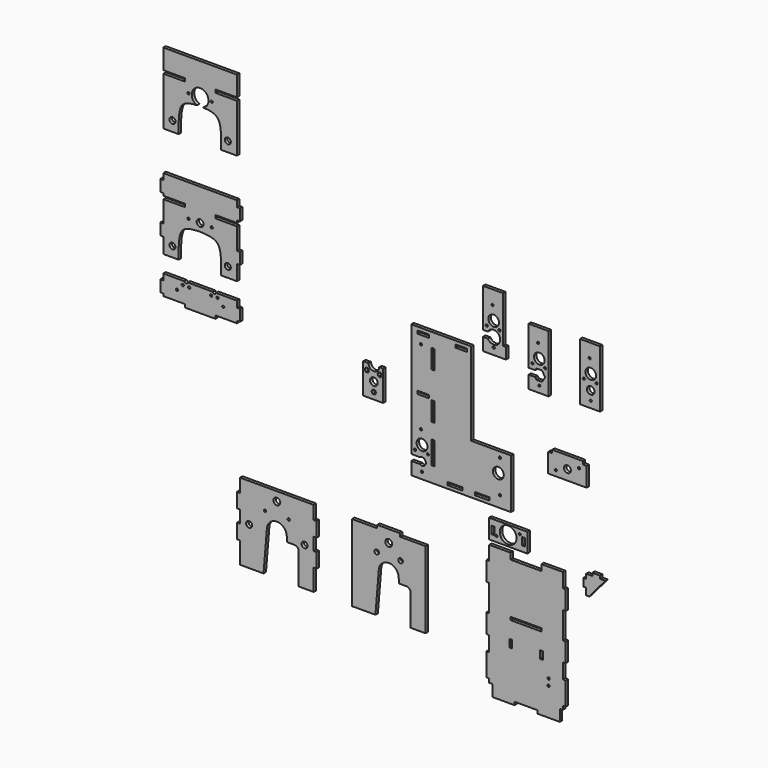
from build123d import *

# Parameters (mm, degrees)
F0_R      = 1.4
F0_R_2    = 7.1
F0_W      = 3.9
F0_H      = 30
F0_W_2    = 19
F0_H_2    = 3.9
F0_H_3    = 25
F0_R_3    = 1.5
F0_W_3    = 15
F2_DEPTH  = 4
F1_R      = 1.4
F1_R_2    = 4.5
F3_DEPTH  = 4
F4_R      = 1.4
F4_W      = 3.9
F4_H      = 10
F4_R_2    = 10.9
F5_DEPTH  = 4
F7_DEPTH  = 4
F8_W      = 3.7
F8_H      = 10
F8_R      = 1.5
F8_W_2    = 40
F8_H_2    = 3.9
F9_DEPTH  = 4
F10_R     = 1.4
F10_R_2   = 6.95
F11_DEPTH = 4
F12_R     = 1.5
F12_R_2   = 1.4
F12_R_3   = 6.95
F13_DEPTH = 4
F14_R     = 1.4
F14_R_2   = 5
F14_R_3   = 6.95
F15_DEPTH = 4
F16_R     = 5
F17_DEPTH = 4
F18_R     = 3
F18_R_2   = 4.5
F19_DEPTH = 4
F20_R     = 3.925
F20_R_2   = 1.5
F20_R_3   = 4.5
F21_DEPTH = 4
F22_R     = 1.45
F22_R_2   = 1.5
F23_DEPTH = 4
F24_R     = 3.925
F24_R_2   = 1.4
F24_R_3   = 4.5
F25_DEPTH = 4
F26_R     = 3.925
F26_R_2   = 1.4
F27_DEPTH = 4


# Not quite as in the source:
# - ends of sketch curves that miss each other by under 0.0002 mm in the source are joined
# - the dataset's text gives a spline's control points without its knots; the knots are read off the source's solid


with BuildPart() as f2:
    # F0 (on Front) → F2 (new body)
    with BuildSketch(Plane.XZ):
        with BuildLine():
            Line((-63.4341964287, 90.4360366771), (-63.4341964287, -22.9460053229))
            Line((-63.4341964287, -22.9460053229), (-63.4341964287, -58.4452043229))
            Line((-63.4341964287, -58.4452043229), (-52.4341964287, -58.4452043229))
            ThreePointArc((-52.4341964287, -58.4452043229), (-47.1981284512, -57.9730683679), (-44.4341964287, -62.4452043229))
            ThreePointArc((-44.4341964287, -62.4452043229), (-47.1981284512, -66.9173402779), (-52.4341964287, -66.4452043229))
            Line((-52.4341964287, -66.4452043229), (-63.4341964287, -66.4452043229))
            Line((-63.4341964287, -66.4452043229), (-63.4341964287, -82.9460053229))
            Line((-63.4341964287, -82.9460053229), (66.5658035713, -82.9460053229))
            Line((66.5658035713, -82.9460053229), (66.5629615713, -50.5350533229))
            Line((66.5629615713, -50.5350533229), (66.5658035713, -17.9460053229))
            Line((66.5658035713, -17.9460053229), (29.5658035713, -17.9460053229))
            Line((29.5658035713, -17.9460053229), (19.5658035713, -17.9460053229))
            Line((19.5658035713, -17.9460053229), (14.5658035713, -17.9460053229))
            Line((14.5658035713, -17.9460053229), (14.5658035713, 90.4360366771))
            Line((14.5658035713, 90.4360366771), (-63.4341964287, 90.4360366771))
        make_face()
        with Locations((-49.4341964287, -74.3492573229)):
            Circle(F0_R, mode=Mode.SUBTRACT)
        with Locations((-58.4986314287, -51.9228453229)):
            Circle(F0_R, mode=Mode.SUBTRACT)
        with Locations((-49.4341964287, -43.4452043229)):
            Circle(F0_R_2, mode=Mode.SUBTRACT)
        with Locations((-41.8097264287, -51.9228453229)):
            Circle(F0_R, mode=Mode.SUBTRACT)
        with Locations((-35.4341964287, -47.9460053229)):
            Rectangle(F0_W, F0_H, mode=Mode.SUBTRACT)
        with Locations((-6.4341964287, -76.9460053229)):
            Rectangle(F0_W_2, F0_H_2, mode=Mode.SUBTRACT)
        with Locations((-50.9341964287, -25.9460053229)):
            Circle(F0_R, mode=Mode.SUBTRACT)
        with Locations((-35.4341964287, -0.4460053229)):
            Rectangle(F0_W, F0_H_3, mode=Mode.SUBTRACT)
        with Locations((29.0658035713, -76.9460053229)):
            Rectangle(F0_W_2, F0_H_2, mode=Mode.SUBTRACT)
        with Locations((52.2136285713, -67.9460053229)):
            Circle(F0_R_3, mode=Mode.SUBTRACT)
        with Locations((50.0757545713, -43.5444653229)):
            Circle(F0_R_2, mode=Mode.SUBTRACT)
        with Locations((52.2136285713, -24.9473123229)):
            Circle(F0_R_3, mode=Mode.SUBTRACT)
        with Locations((-47.9341964287, 14.9539946771)):
            Rectangle(F0_W_3, F0_H_2, mode=Mode.SUBTRACT)
        with Locations((-35.4341964287, 59.5539946771)):
            Rectangle(F0_W, F0_H_3, mode=Mode.SUBTRACT)
        with Locations((-50.9341964287, 71.6313536771)):
            Circle(F0_R, mode=Mode.SUBTRACT)
        with Locations((-47.9341964287, 84.2463486771)):
            Rectangle(F0_W_3, F0_H_2, mode=Mode.SUBTRACT)
        with Locations((1.9138515713, 84.2463486771)):
            Rectangle(F0_W_3, F0_H_2, mode=Mode.SUBTRACT)
    extrude(amount=F2_DEPTH)


with BuildPart() as f3:
    # F1 (on Front) → F3 (new body)
    with BuildSketch(Plane.XZ):
        Polygon((115.1583404474, -22.8264850692), (120.1583404474, -22.8264850692), (160.1583404474, -22.8264850692), (165.1583404474, -22.8264850692), (165.1583404474, 2.1735149308), (162.1583404474, 2.1735149308), (160.1583404474, 2.1735149308), (160.1583404474, 6.1735149308), (120.1583404474, 6.1735149308), (120.1583404474, 2.1735149308), (118.1583404474, 2.1735149308), (115.1583404474, 2.1735149308), (115.1583404474, -9.8264850692), align=None)
        with Locations((124.9870464474, -15.6336020692)):
            Circle(F1_R, mode=Mode.SUBTRACT)
        with Locations((140.1583404474, -9.6756990692)):
            Circle(F1_R_2, mode=Mode.SUBTRACT)
        with Locations((155.3296344474, -3.7691630692)):
            Circle(F1_R, mode=Mode.SUBTRACT)
    extrude(amount=F3_DEPTH)


with BuildPart() as f5:
    # F4 (on Front) → F5 (new body)
    with BuildSketch(Plane.XZ):
        Polygon((82.8902986646, -98.5648238522), (42.8902986646, -98.5648238522), (37.8902986646, -98.5648238522), (37.8902986646, -110.5648238522), (37.8902986646, -123.5648238522), (42.8902986646, -123.5648238522), (82.8902986646, -123.5648238522), (87.8902986646, -123.5648238522), (87.8902986646, -110.5648238522), (87.8902986646, -98.5648238522), align=None)
        with Locations((47.7190046646, -116.3719408522)):
            Circle(F4_R, mode=Mode.SUBTRACT)
        with Locations((42.9902986646, -111.5648238522)):
            Rectangle(F4_W, F4_H, mode=Mode.SUBTRACT)
        with Locations((82.7902986646, -111.5648238522)):
            Rectangle(F4_W, F4_H, mode=Mode.SUBTRACT)
        with Locations((62.8902986646, -110.4140378522)):
            Circle(F4_R_2, mode=Mode.SUBTRACT)
        with Locations((78.0615926646, -104.5075018522)):
            Circle(F4_R, mode=Mode.SUBTRACT)
    extrude(amount=F5_DEPTH)


with BuildPart() as f7:
    # F6 (on Front) → F7 (new body)
    with BuildSketch(Plane.XZ):
        Polygon((164.545552, -137.732495), (164.545552, -146.610202), (168.63066, -146.610202), (189.545552, -121.732495), (182.545552, -121.732495), (182.545552, -118.032495), (172.545552, -118.032495), (172.545552, -121.732495), (164.545552, -121.732495), (164.545552, -127.732495), (160.845552, -127.732495), (160.845552, -137.732495), align=None)
    extrude(amount=F7_DEPTH)


with BuildPart() as f9:
    # F8 (on Front) → F9 (new body)
    with BuildSketch(Plane.XZ):
        Polygon((134.185844, -129.659568), (106.185844, -129.659568), (106.185844, -137.659568), (66.185844, -137.659568), (66.185844, -129.659568), (38.185844, -129.659568), (38.185844, -148.305989), (34.485844, -148.305989), (34.485844, -173.305989), (38.185844, -173.305989), (38.185844, -208.305989), (34.485844, -208.305989), (34.485844, -233.305989), (38.185844, -233.305989), (38.185844, -253.04161), (34.485844, -253.04161), (34.485844, -283.04161), (38.185844, -283.04161), (38.185844, -288.04161), (42.185844, -288.04161), (42.185844, -303.04161), (71.185844, -303.04161), (71.185844, -299.04161), (101.185844, -299.04161), (101.185844, -303.04161), (130.185844, -303.04161), (130.185844, -288.04161), (134.185844, -288.04161), (134.185844, -283.04161), (137.885844, -283.04161), (137.885844, -253.04161), (134.185844, -253.04161), (134.185844, -233.305989), (137.885844, -233.305989), (137.885844, -208.305989), (134.185844, -208.305989), (134.185844, -173.305989), (137.885844, -173.305989), (137.885844, -148.305989), (134.185844, -148.305989), align=None)
        with Locations((66.166966, -234.041521)):
            Rectangle(F8_W, F8_H, mode=Mode.SUBTRACT)
        with Locations((115.552706, -266.295691)):
            Circle(F8_R, mode=Mode.SUBTRACT)
        Polygon((108.016966, -229.041521), (108.016966, -239.041521), (104.316966, -239.041521), (104.316966, -229.084858), (104.316966, -229.041521), align=None, mode=Mode.SUBTRACT)
        with Locations((115.552706, -257.951092)):
            Circle(F8_R, mode=Mode.SUBTRACT)
        with Locations((86.185844, -205.14161)):
            Rectangle(F8_W_2, F8_H_2, mode=Mode.SUBTRACT)
    extrude(amount=F9_DEPTH)


with BuildPart() as f11:
    # F10 (on Front) → F11 (new body)
    with BuildSketch(Plane.XZ):
        Polygon((89.4677672969, 81.3291730556), (89.4677672969, 65.8326860556), (115.5677672969, 65.8326860556), (115.5677672969, 140.8326860556), (89.4677672969, 140.8326860556), (89.4677672969, 90.3228060556), (98.2716152969, 90.3228060556), (99.7149902969, 92.8228060556), (107.2205442969, 92.8228060556), (110.9733212969, 86.3228060556), (107.2205442969, 79.8228060556), (99.7149902969, 79.8228060556), (98.2716150084, 82.322805889), (89.4677672969, 82.3228060556), align=None)
        with Locations((94.4033322969, 96.8451650556)):
            Circle(F10_R, mode=Mode.SUBTRACT)
        with Locations((103.4677672969, 74.4187530556)):
            Circle(F10_R, mode=Mode.SUBTRACT)
        with Locations((111.0922382969, 96.8451650556)):
            Circle(F10_R, mode=Mode.SUBTRACT)
        with Locations((101.9677672969, 122.8326860556)):
            Circle(F10_R, mode=Mode.SUBTRACT)
        with Locations((103.4677672969, 105.3228060556)):
            Circle(F10_R_2, mode=Mode.SUBTRACT)
    extrude(amount=F11_DEPTH)


with BuildPart() as f13:
    # F12 (on Front) → F13 (new body)
    with BuildSketch(Plane.XZ):
        with BuildLine():
            Line((30.0127932642, 106.5112202716), (30.0127932642, 90.0211002716))
            Line((30.0127932642, 90.0211002716), (60.0127932642, 90.0211002716))
            Line((60.0127932642, 90.0211002716), (60.0127932642, 104.5211002716))
            Line((60.0127932642, 104.5211002716), (56.1127932642, 104.5211002716))
            Line((56.1127932642, 104.5211002716), (56.1127932642, 165.0211002716))
            Line((56.1127932642, 165.0211002716), (30.0127932642, 165.0211002716))
            Line((30.0127932642, 165.0211002716), (30.0127932642, 114.5112202716))
            Line((30.0127932642, 114.5112202716), (36.5127932642, 114.5112202716))
            ThreePointArc((36.5127932642, 114.5112202716), (46.0743460771, 118.7574315228), (52.5127932642, 110.5112202716))
            ThreePointArc((52.5127932642, 110.5112202716), (46.0743460771, 102.2650090204), (36.5127932642, 106.5112202716))
            Line((36.5127932642, 106.5112202716), (30.0127932642, 106.5112202716))
        make_face()
        with Locations((44.0127932642, 98.6071672716)):
            Circle(F12_R, mode=Mode.SUBTRACT)
        with Locations((34.9483582642, 121.0335792716)):
            Circle(F12_R_2, mode=Mode.SUBTRACT)
        with Locations((44.0127932642, 129.5112202716)):
            Circle(F12_R_3, mode=Mode.SUBTRACT)
        with Locations((42.5127932642, 147.0211002716)):
            Circle(F12_R_2, mode=Mode.SUBTRACT)
        with Locations((51.6372632642, 121.0335792716)):
            Circle(F12_R_2, mode=Mode.SUBTRACT)
    extrude(amount=F13_DEPTH)


with BuildPart() as f15:
    # F14 (on Front) → F15 (new body)
    with BuildSketch(Plane.XZ):
        Polygon((156.5812625652, 109.6729690981), (156.5812625652, 70.1828490981), (182.6812625652, 70.1828490981), (182.6812625652, 84.6828490981), (182.6812625652, 109.6729690981), (182.6812625652, 145.1828490981), (156.5812625652, 145.1828490981), align=None)
        with Locations((161.5168275652, 101.1953280981)):
            Circle(F14_R, mode=Mode.SUBTRACT)
        with Locations((170.5812625652, 78.7689160981)):
            Circle(F14_R, mode=Mode.SUBTRACT)
        with Locations((170.5812625652, 90.6729690981)):
            Circle(F14_R_2, mode=Mode.SUBTRACT)
        with Locations((178.2057335652, 101.1953280981)):
            Circle(F14_R, mode=Mode.SUBTRACT)
        with Locations((169.0812625652, 127.1828490981)):
            Circle(F14_R, mode=Mode.SUBTRACT)
        with Locations((170.5812625652, 109.6729690981)):
            Circle(F14_R_3, mode=Mode.SUBTRACT)
    extrude(amount=F15_DEPTH)


with BuildPart() as f17:
    # F16 (on Front) → F17 (new body)
    with BuildSketch(Plane.XZ):
        with BuildLine():
            Line((-126.2313253517, 27.6353715188), (-126.2313253517, -11.8547484812))
            Line((-126.2313253517, -11.8547484812), (-100.1313253517, -11.8547484812))
            Line((-100.1313253517, -11.8547484812), (-100.1313253517, 27.6353715188))
            Line((-100.1313253517, 27.6353715188), (-105.2813253517, 27.6353715188))
            ThreePointArc((-105.2813253517, 27.6353715188), (-112.2313253517, 20.6853715188), (-119.1813253517, 27.6353715188))
            Line((-119.1813253517, 27.6353715188), (-126.2313253517, 27.6353715188))
        make_face()
        Polygon((-113.7540863517, -0.6311814812), (-110.7085633517, -0.6311814812), (-109.1858023517, -3.2686814812), (-110.7085633517, -5.9061814812), (-113.7540863517, -5.9061814812), (-115.2768473517, -3.2686814812), align=None, mode=Mode.SUBTRACT)
        Polygon((-122.8185213517, 21.7952305188), (-119.7729983517, 21.7952305188), (-118.2502373517, 19.1577305188), (-119.7729983517, 16.5202305188), (-122.8185213517, 16.5202305188), (-124.3412823517, 19.1577305188), align=None, mode=Mode.SUBTRACT)
        with Locations((-112.2313253517, 8.6353715188)):
            Circle(F16_R, mode=Mode.SUBTRACT)
        Polygon((-106.1296163517, 21.7952305188), (-103.0840933517, 21.7952305188), (-101.5613323517, 19.1577305188), (-103.0840933517, 16.5202305188), (-106.1296163517, 16.5202305188), (-107.6523773517, 19.1577305188), align=None, mode=Mode.SUBTRACT)
    extrude(amount=F17_DEPTH)


with BuildPart() as f19:
    # F18 (on Front) → F19 (new body)
    with BuildSketch(Plane.XZ):
        with BuildLine():
            Line((-107.860674, -158.209543), (-140.860674, -158.209543))
            Line((-140.860674, -158.209543), (-140.860674, -229.734601))
            Line((-140.860674, -229.734601), (-140.860674, -230.734601))
            Line((-140.860674, -230.734601), (-140.860674, -258.260348))
            Line((-140.860674, -258.260348), (-110.19947, -258.260348))
            Line((-110.19947, -258.260348), (-105.8603875582, -205.9732646507))
            ThreePointArc((-105.8603875582, -205.9732646507), (-92.860673958, -193.059563), (-79.8609604413, -205.9732647348))
            Line((-79.8609604413, -205.9732647348), (-79.33473, -212.314486))
            Line((-79.33473, -212.314486), (-70.172244, -212.314486))
            ThreePointArc((-70.172244, -212.314486), (-66.000313991, -214.042555991), (-64.272244, -218.214486))
            Line((-64.272244, -218.214486), (-64.272244, -258.260348))
            Line((-64.272244, -258.260348), (-44.860674, -258.260348))
            Line((-44.860674, -258.260348), (-44.860674, -230.734601))
            Line((-44.860674, -230.734601), (-44.860674, -229.734601))
            Line((-44.860674, -229.734601), (-44.860674, -158.209543))
            Line((-44.860674, -158.209543), (-77.860674, -158.209543))
            Line((-77.860674, -158.209543), (-77.860674, -154.209543))
            Line((-77.860674, -154.209543), (-107.860674, -154.209543))
            Line((-107.860674, -154.209543), (-107.860674, -158.209543))
        make_face()
        with Locations((-108.360674, -185.559563)):
            Circle(F18_R, mode=Mode.SUBTRACT)
        with Locations((-92.860674, -170.059563)):
            Circle(F18_R_2, mode=Mode.SUBTRACT)
        with Locations((-77.360674, -185.559563)):
            Circle(F18_R, mode=Mode.SUBTRACT)
    extrude(amount=F19_DEPTH)


with BuildPart() as f21:
    # F20 (on Front) → F21 (new body)
    with BuildSketch(Plane.XZ):
        with BuildLine():
            Line((-290.77723, -194.760348), (-286.77723, -194.760348))
            Line((-286.77723, -194.760348), (-286.77723, -211.260348))
            Line((-286.77723, -211.260348), (-290.77723, -211.260348))
            Line((-290.77723, -211.260348), (-290.77723, -230.260348))
            Line((-290.77723, -230.260348), (-286.77723, -230.260348))
            Line((-286.77723, -230.260348), (-286.77723, -258.260348))
            Line((-286.77723, -258.260348), (-256.116026, -258.260348))
            Line((-256.116026, -258.260348), (-251.7769435582, -205.9732646507))
            ThreePointArc((-251.7769435582, -205.9732646507), (-238.777229958, -193.059563), (-225.7775164413, -205.9732647348))
            Line((-225.7775164413, -205.9732647348), (-225.251286, -212.314486))
            Line((-225.251286, -212.314486), (-216.0888, -212.314486))
            ThreePointArc((-216.0888, -212.314486), (-211.916869991, -214.042555991), (-210.1888, -218.214486))
            Line((-210.1888, -218.214486), (-210.1888, -258.260348))
            Line((-210.1888, -258.260348), (-190.77723, -258.260348))
            Line((-190.77723, -258.260348), (-190.77723, -230.260348))
            Line((-190.77723, -230.260348), (-186.77723, -230.260348))
            Line((-186.77723, -230.260348), (-186.77723, -211.260348))
            Line((-186.77723, -211.260348), (-190.77723, -211.260348))
            Line((-190.77723, -211.260348), (-190.77723, -194.760348))
            Line((-190.77723, -194.760348), (-186.77723, -194.760348))
            Line((-186.77723, -194.760348), (-186.77723, -175.760348))
            Line((-186.77723, -175.760348), (-190.77723, -175.760348))
            Line((-190.77723, -175.760348), (-190.77723, -158.209543))
            Line((-190.77723, -158.209543), (-286.77723, -158.209543))
            Line((-286.77723, -158.209543), (-286.77723, -175.760348))
            Line((-286.77723, -175.760348), (-290.77723, -175.760348))
            Line((-290.77723, -175.760348), (-290.77723, -194.760348))
        make_face()
        with Locations((-274.87723, -208.059563)):
            Circle(F20_R, mode=Mode.SUBTRACT)
        with Locations((-254.27723, -185.559563)):
            Circle(F20_R_2, mode=Mode.SUBTRACT)
        with Locations((-238.77723, -170.059563)):
            Circle(F20_R_3, mode=Mode.SUBTRACT)
        with Locations((-223.27723, -185.559563)):
            Circle(F20_R_2, mode=Mode.SUBTRACT)
        with Locations((-202.677233, -208.058757)):
            Circle(F20_R, mode=Mode.SUBTRACT)
    extrude(amount=F21_DEPTH)


with BuildPart() as f23:
    # F22 (on Front) → F23 (new body)
    with BuildSketch(Plane.XZ):
        with BuildLine():
            Line((-359.253564, 43.629415), (-386.77723, 43.629415))
            Line((-386.77723, 43.629415), (-386.77723, 35.629415))
            Line((-386.77723, 35.629415), (-390.77723, 35.629415))
            Line((-390.77723, 35.629415), (-390.77723, 20.629415))
            Line((-390.77723, 20.629415), (-386.77723, 20.629415))
            Line((-386.77723, 20.629415), (-386.77723, 17.629415))
            Line((-386.77723, 17.629415), (-358.77723, 17.629415))
            Line((-358.77723, 17.629415), (-358.77723, 13.629415))
            Line((-358.77723, 13.629415), (-318.77723, 13.629415))
            Line((-318.77723, 13.629415), (-318.77723, 17.629415))
            Line((-318.77723, 17.629415), (-290.77723, 17.629415))
            Line((-290.77723, 17.629415), (-290.77723, 20.629415))
            Line((-290.77723, 20.629415), (-286.77723, 20.629415))
            Line((-286.77723, 20.629415), (-286.77723, 35.629415))
            Line((-286.77723, 35.629415), (-290.77723, 35.629415))
            Line((-290.77723, 35.629415), (-290.77723, 43.629415))
            Line((-290.77723, 43.629415), (-318.300896, 43.629415))
            ThreePointArc((-318.300896, 43.629415), (-320.300896, 41.629415), (-322.300896, 43.629415))
            Line((-322.300896, 43.629415), (-355.253564, 43.629415))
            ThreePointArc((-355.253564, 43.629415), (-357.253564, 41.629415), (-359.253564, 43.629415))
        make_face()
        with Locations((-368.982704, 30.877128)):
            Circle(F22_R, mode=Mode.SUBTRACT)
        with Locations((-361.425863, 38.520697)):
            Circle(F22_R_2, mode=Mode.SUBTRACT)
        with Locations((-353.081264, 38.520697)):
            Circle(F22_R_2, mode=Mode.SUBTRACT)
        with Locations((-308.571756, 30.877128)):
            Circle(F22_R, mode=Mode.SUBTRACT)
        with Locations((-324.473196, 38.520697)):
            Circle(F22_R_2, mode=Mode.SUBTRACT)
        with Locations((-316.128597, 38.520697)):
            Circle(F22_R_2, mode=Mode.SUBTRACT)
    extrude(amount=F23_DEPTH)


with BuildPart() as f25:
    # F24 (on Front) → F25 (new body)
    with BuildSketch(Plane.XZ):
        with BuildLine():
            Line((-290.77723, 128.899888), (-292.77723, 128.899888))
            Line((-292.77723, 128.899888), (-318.77723, 128.899888))
            Line((-318.77723, 128.899888), (-318.77723, 132.899888))
            Line((-318.77723, 132.899888), (-290.77723, 132.899888))
            Line((-290.77723, 132.899888), (-290.77723, 135.899888))
            Line((-290.77723, 135.899888), (-286.77723, 135.899888))
            Line((-286.77723, 135.899888), (-286.77723, 150.899888))
            Line((-286.77723, 150.899888), (-290.77723, 150.899888))
            Line((-290.77723, 150.899888), (-290.77723, 158.899888))
            Line((-290.77723, 158.899888), (-386.77723, 158.899888))
            Line((-386.77723, 158.899888), (-386.77723, 150.899888))
            Line((-386.77723, 150.899888), (-390.77723, 150.899888))
            Line((-390.77723, 150.899888), (-390.77723, 135.899888))
            Line((-390.77723, 135.899888), (-386.77723, 135.899888))
            Line((-386.77723, 135.899888), (-386.77723, 132.899888))
            Line((-386.77723, 132.899888), (-358.77723, 132.899888))
            Line((-358.77723, 132.899888), (-358.77723, 128.899888))
            Line((-358.77723, 128.899888), (-384.77723, 128.899888))
            Line((-384.77723, 128.899888), (-386.77723, 128.899888))
            Line((-386.77723, 128.899888), (-386.77723, 108.899888))
            Line((-386.77723, 108.899888), (-386.77723, 100.899888))
            Line((-386.77723, 100.899888), (-390.77723, 100.899888))
            Line((-390.77723, 100.899888), (-390.77723, 85.899888))
            Line((-390.77723, 85.899888), (-386.77723, 85.899888))
            Line((-386.77723, 85.899888), (-386.77723, 65.899888))
            Line((-386.77723, 65.899888), (-366.77723, 65.899888))
            Line((-366.77723, 65.899888), (-366.77723, 80.051479))
            add(Edge.make_bspline(
                [(-366.77723, 80.051479), (-366.29799, 88.643119), (-365.399503, 104.750867), (-350.190306, 106.459967), (-342.731447, 106.893205)],
                knots=[0, 0, 0, 0, 22.367563, 41.935074, 41.935074, 41.935074, 41.935074], degree=3))
            Line((-342.731447, 106.893205), (-339.27723, 107.051479))
            Line((-339.27723, 107.051479), (-338.27723, 107.051479))
            add(Edge.make_bspline(
                [(-311.27723, 80.051479), (-311.75647, 88.643119), (-312.710073, 105.738961), (-329.783953, 106.615468), (-338.27723, 107.051479)],
                knots=[0, 0, 0, 0, 22.367563, 44.507488, 44.507488, 44.507488, 44.507488], degree=3))
            Line((-311.27723, 80.051479), (-311.27723, 65.899888))
            Line((-311.27723, 65.899888), (-290.77723, 65.899888))
            Line((-290.77723, 65.899888), (-290.77723, 85.899888))
            Line((-290.77723, 85.899888), (-286.77723, 85.899888))
            Line((-286.77723, 85.899888), (-286.77723, 100.899888))
            Line((-286.77723, 100.899888), (-290.77723, 100.899888))
            Line((-290.77723, 100.899888), (-290.77723, 108.899888))
            Line((-290.77723, 108.899888), (-290.77723, 128.899888))
        make_face()
        with Locations((-374.877227, 79.051479)):
            Circle(F24_R, mode=Mode.SUBTRACT)
        with Locations((-302.67723, 79.050674)):
            Circle(F24_R, mode=Mode.SUBTRACT)
        with Locations((-353.948524, 117.050674)):
            Circle(F24_R_2, mode=Mode.SUBTRACT)
        with Locations((-338.77723, 117.050674)):
            Circle(F24_R_3, mode=Mode.SUBTRACT)
        with Locations((-323.605936, 117.050674)):
            Circle(F24_R_2, mode=Mode.SUBTRACT)
    extrude(amount=F25_DEPTH)


with BuildPart() as f27:
    # F26 (on Front) → F27 (new body)
    with BuildSketch(Plane.XZ):
        with BuildLine():
            ThreePointArc((-342.7314468574, 251.0349273663), (-338.7415971881, 272.0923377568), (-334.8895081602, 251.0092914196))
            add(Edge.make_bspline(
                [(-311.27723, 224.193201), (-311.75647, 232.784841), (-312.646827, 248.746834), (-327.590078, 250.56958), (-334.8895081602, 251.0092914196)],
                knots=[0, 0, 0, 0, 22.367563, 41.555614, 41.555614, 41.555614, 41.555614], degree=3))
            Line((-311.27723, 224.193201), (-311.27723, 210.04161))
            Line((-311.27723, 210.04161), (-299.77723, 210.04161))
            Line((-299.77723, 210.04161), (-290.77723, 210.04161))
            Line((-290.77723, 210.04161), (-290.77723, 273.04161))
            Line((-290.77723, 273.04161), (-292.77723, 273.04161))
            Line((-292.77723, 273.04161), (-318.77723, 273.04161))
            Line((-318.77723, 273.04161), (-318.77723, 277.04161))
            Line((-318.77723, 277.04161), (-290.77723, 277.04161))
            Line((-290.77723, 277.04161), (-290.77723, 303.04161))
            Line((-290.77723, 303.04161), (-386.77723, 303.04161))
            Line((-386.77723, 303.04161), (-386.77723, 277.04161))
            Line((-386.77723, 277.04161), (-358.77723, 277.04161))
            Line((-358.77723, 277.04161), (-358.77723, 273.04161))
            Line((-358.77723, 273.04161), (-384.77723, 273.04161))
            Line((-384.77723, 273.04161), (-386.77723, 273.04161))
            Line((-386.77723, 273.04161), (-386.77723, 210.04161))
            Line((-386.77723, 210.04161), (-377.77723, 210.04161))
            Line((-377.77723, 210.04161), (-366.77723, 210.04161))
            Line((-366.77723, 210.04161), (-366.77723, 224.193201))
            add(Edge.make_bspline(
                [(-366.77723, 224.193201), (-366.29799, 232.784841), (-365.399503, 248.892589), (-350.190306, 250.601689), (-342.7314468574, 251.0349273663)],
                knots=[0, 0, 0, 0, 22.367563, 41.935074, 41.935074, 41.935074, 41.935074], degree=3))
        make_face()
        with Locations((-374.877227, 223.193201)):
            Circle(F26_R, mode=Mode.SUBTRACT)
        with Locations((-302.67723, 223.192396)):
            Circle(F26_R, mode=Mode.SUBTRACT)
        with Locations((-353.948524, 261.192396)):
            Circle(F26_R_2, mode=Mode.SUBTRACT)
        with Locations((-323.605936, 261.192396)):
            Circle(F26_R_2, mode=Mode.SUBTRACT)
    extrude(amount=F27_DEPTH)


solid = Compound([f2.part, f3.part, f5.part, f7.part, f9.part, f11.part, f13.part, f15.part, f17.part, f19.part, f21.part, f23.part, f25.part, f27.part])
